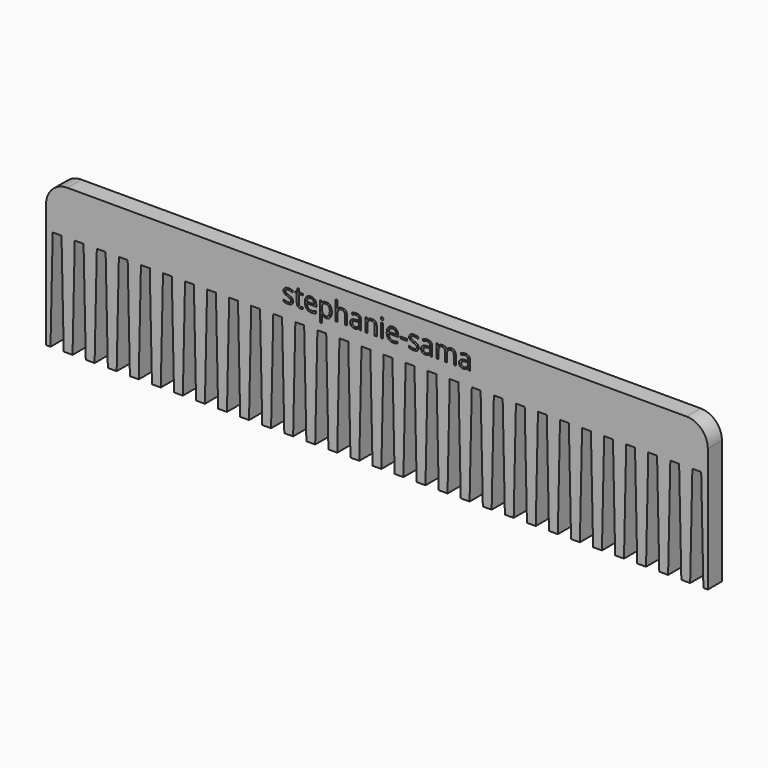
from build123d import *

# Parameters (mm, degrees)
F1_DEPTH     = 4
F2_R         = 4.8284271247
F4_TEXT_SIZE = 5.7827326331
F5_DEPTH     = 1


# Not quite as in the source:
# - Text() gives the source's letters only with a copy of the font that has no kerning and outlines rounded to 1/6400 em; it was checked with that copy


with BuildPart() as f1:
    # F0 (on Front) → F1 (new body)
    with BuildSketch(Plane.XZ):
        Polygon((0, 32.9804583299), (0, 0), (1, 0), (1.5, 22.9945645751), (3.5, 22.9945645751), (4, 0), (6, 0), (6.5, 22.9945645751), (8.5, 22.9945645751), (9, 0), (11, 0), (11.5, 22.9945645751), (13.5, 22.9945645751), (14, 0), (16, 0), (16.5, 22.9945645751), (18.5, 22.9945645751), (19, 0), (21, 0), (21.5, 22.9945645751), (23.5, 22.9945645751), (24, 0), (26, 0), (26.5, 22.9945645751), (28.5, 22.9945645751), (29, 0), (31, 0), (31.5, 22.9945645751), (33.5, 22.9945645751), (34, 0), (36, 0), (36.5, 22.9945645751), (38.5, 22.9945645751), (39, 0), (41, 0), (41.5, 22.9945645751), (43.5, 22.9945645751), (44, 0), (46, 0), (46.5, 22.9945645751), (48.5, 22.9945645751), (49, 0), (51, 0), (51.5, 22.9945645751), (53.5, 22.9945645751), (54, 0), (56, 0), (56.5, 22.9945645751), (58.5, 22.9945645751), (59, 0), (61, 0), (61.5, 22.9945645751), (63.5, 22.9945645751), (64, 0), (66, 0), (66.5, 22.9945645751), (68.5, 22.9945645751), (69, 0), (71, 0), (71.5, 22.9945645751), (73.5, 22.9945645751), (74, 0), (75, 0), (75, 32.9804583299), align=None)
    extrude(amount=F1_DEPTH)

    # F2
    f2_edges = [f1.edges().sort_by_distance(p)[0] for p in [
        (75, -2, 32.980458),
    ]]
    fillet(f2_edges, radius=F2_R)

    # F3: F1 across plane


with BuildPart() as f1_1:
    add(f1.part)
    add(f1.part.mirror(Plane.YZ))

    # F4 (on face) → F5 (cut)
    with BuildSketch(Plane.XZ.offset(4)):
        with Locations((-21.4729126601, 26.1033866554)):
            Text('stephanie-sama', F4_TEXT_SIZE, font='Open Sans', text_align=(TextAlign.LEFT, TextAlign.BOTTOM))
    extrude(amount=-F5_DEPTH, mode=Mode.SUBTRACT)


solid = f1_1.part
